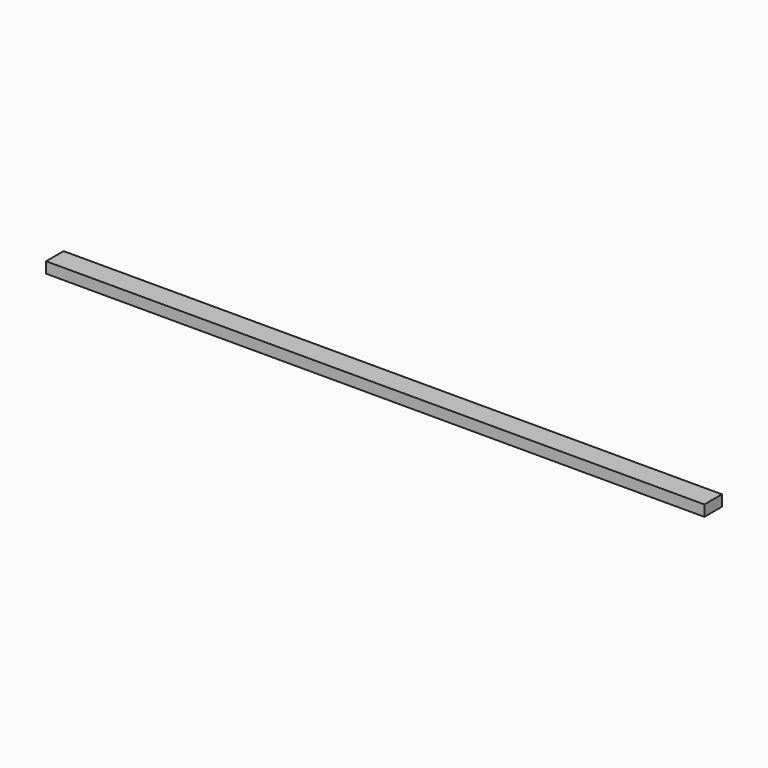
from build123d import *

# Parameters (mm, degrees)
F0_W     = 1524
F0_H     = 50.8
F1_DEPTH = 25.4


# Not quite as in the source:
# - a feature names something its author has since deleted; it is built from what else it names


with BuildPart() as f1:
    # F0 (on Top) → F1 (new body)
    with BuildSketch(Plane.XY):
        with Locations((762, 25.4)):
            Rectangle(F0_W, F0_H)
    extrude(amount=F1_DEPTH)


solid = f1.part
